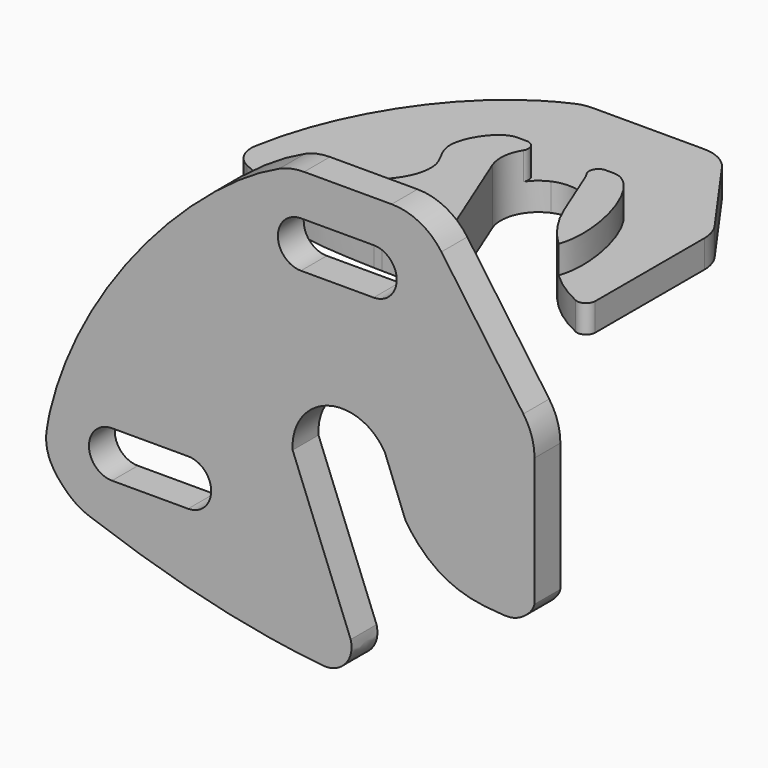
from build123d import *

# Parameters (mm, degrees)
F1_DEPTH    = 3
F2_DEPTH    = 6
F3_T1_DEPTH = 9.5721041615
F3_T3_DEPTH = 10.6008199663
F3_T5_DEPTH = 13.4715090396
F5_DEPTH    = 3.5
F6_R        = 6.6


# Not quite as in the source:
# - a fillet or chamfer that OpenCascade refuses, or shapes differently, is made with other operations: its cross-section is extruded or revolved along the edge and cut away or added


with BuildPart() as f1:
    # F0 (on Top) → F1 (new body)
    with BuildSketch(Plane.XY):
        with BuildLine():
            Line((10.45310308, 40.5577271794), (4.2537174463, 49.2922064861))
            ThreePointArc((4.2537174463, 49.2922064861), (2.8274809851, 50.5309572011), (0.9918162896, 50.9770389232))
            Line((0.9918162896, 50.9770389232), (-11.1394110977, 50.9770389232))
            ThreePointArc((-11.1394110977, 50.9770389232), (-11.971760899, 50.8894798248), (-12.7676708013, 50.6306358273))
            add(Edge.make_bspline(
                [(-29.0087616808, 27.7205901484), (-27.4187770892, 36.9581566811), (-21.4067194111, 46.7805628451), (-12.7676708013, 50.6306358273)],
                knots=[2.2635349129, 2.2635349129, 2.2635349129, 2.2635349129, 29.9811081227, 29.9811081227, 29.9811081227, 29.9811081227], degree=3))
            ThreePointArc((-29.0087616808, 27.7205901484), (-28.7134700585, 25.8268482821), (-27.3319649166, 24.4983532911))
            add(Edge.make_bspline(
                [(-27.3319649166, 24.4983532911), (-21.9405178356, 21.9555285826), (-18.2546260968, 21.2787347002), (-10.8634286016, 21.0598215648)],
                knots=[2.2151277371, 2.2151277371, 2.2151277371, 2.2151277371, 21.0948867648, 21.0948867648, 21.0948867648, 21.0948867648], degree=3))
            ThreePointArc((-10.8634286016, 21.0598215648), (-13.1384704579, 22.9593681642), (-12.6555627212, 25.8835591376))
            add(Edge.make_bspline(
                [(-8.9445100778, 38.260217756), (-10.7857445501, 38.3745139324), (-13.9860512104, 33.4519520511), (-10.6280428717, 30.4447296599), (-11.5734467469, 27.2133998528), (-12.6555627212, 25.8835591376)],
                knots=[0, 0, 0, 0, 0.371058298, 0.6724870623, 1, 1, 1, 1], degree=3))
            Line((-8.9445100778, 38.260217756), (-5.4481702034, 38.260217756))
            ThreePointArc((-5.4481702034, 38.260217756), (-3.7885215093, 38.6125725889), (-2.1288728152, 38.260217756))
            Line((-2.1288728152, 38.260217756), (1.3674670593, 38.260217756))
            add(Edge.make_bspline(
                [(5.8108489029, 25.2381619066), (7.2972377823, 29.2682433996), (4.5647696354, 38.260217756), (1.3674670593, 38.260217756)],
                knots=[0, 0, 0, 0, 13.7592725372, 13.7592725372, 13.7592725372, 13.7592725372], degree=3))
            ThreePointArc((5.8108489029, 25.2381619066), (8.3264404263, 23.3377486264), (11.1912019233, 22.0213471249))
            Line((11.1912019233, 22.0213471249), (11.1912019233, 38.2425596166))
            ThreePointArc((11.1912019233, 38.2425596166), (11.0022125915, 39.4575483765), (10.45310308, 40.5577271794))
        make_face()
    extrude(amount=F1_DEPTH)

    # F0 (on Top) → F2 (join)
    with BuildSketch(Plane.XY):
        with BuildLine():
            ThreePointArc((-12.6555627212, 25.8835591376), (-13.1384704579, 22.9593681642), (-10.8634286016, 21.0598215648))
            add(Edge.make_bspline(
                [(-10.8634286016, 21.0598215648), (-10.5727766997, 21.0512130112), (-10.2763949805, 21.0433125162), (-9.9739544094, 21.0360344499)],
                knots=[21.0948867648, 21.0948867648, 21.0948867648, 21.0948867648, 21.8373155625, 21.8373155625, 21.8373155625, 21.8373155625], degree=3))
            add(Edge.make_bspline(
                [(-9.9739544094, 21.0360344499), (-7.8814737991, 20.9856800532), (-5.4989697359, 20.9651199081), (-2.7174725462, 20.9459951911)],
                knots=[21.8373155625, 21.8373155625, 21.8373155625, 21.8373155625, 26.9739209391, 26.9739209391, 26.9739209391, 26.9739209391], degree=3))
            Line((-2.7174725462, 20.9459951911), (-7.5770430185, 33.0005098931))
            ThreePointArc((-7.5770430185, 33.0005098931), (-7.5749144289, 36.0603341373), (-5.4481702034, 38.260217756))
            Line((-5.4481702034, 38.260217756), (-8.9445100778, 38.260217756))
            add(Edge.make_bspline(
                [(-8.9445100778, 38.260217756), (-10.7857445501, 38.3745139324), (-13.9860512104, 33.4519520511), (-10.6280428717, 30.4447296599), (-11.5734467469, 27.2133998528), (-12.6555627212, 25.8835591376)],
                knots=[0, 0, 0, 0, 0.371058298, 0.6724870623, 1, 1, 1, 1], degree=3))
        make_face()
        with BuildLine():
            ThreePointArc((2.274153499, 30.4138629783), (3.7616023103, 27.6340666941), (5.8108489029, 25.2381619066))
            add(Edge.make_bspline(
                [(5.8108489029, 25.2381619066), (7.2972377823, 29.2682433996), (4.5647696354, 38.260217756), (1.3674670593, 38.260217756)],
                knots=[0, 0, 0, 0, 13.7592725372, 13.7592725372, 13.7592725372, 13.7592725372], degree=3))
            Line((1.3674670593, 38.260217756), (-2.1288728152, 38.260217756))
            ThreePointArc((-2.1288728152, 38.260217756), (-0.8497607567, 37.3648907946), (0, 36.0550645915))
            Line((0, 36.0550645915), (2.274153499, 30.4138629783))
        make_face()
    extrude(amount=F2_DEPTH)

    # F3: fillet of radius 1 on 4 edges, made by hand

    # F3_s2 → F3_t1 (cut)
    with BuildSketch(Plane.XY.offset(3)):
        with BuildLine():
            ThreePointArc((0.499968819, 38.260617756), (-0.3772452667, 37.7413074811), (-0.3438640289, 36.7224486062))
            Line((-0.3438640289, 36.7224486062), (-0.4282473137, 36.6686862987))
            ThreePointArc((-0.4282473137, 36.6686862987), (-1.1882692191, 37.5471857074), (-2.1695250121, 38.1687938896))
            Line((-2.1695250121, 38.1687938896), (-2.1288728152, 38.3602723635))
            ThreePointArc((-2.1288728152, 38.3602723635), (-0.8144519981, 38.3602723635), (0.499968819, 38.3606723635))
            Line((0.499968819, 38.3606723635), (0.499968819, 38.260617756))
        make_face()
        with BuildLine():
            ThreePointArc((-7.2331789896, 36.7224486062), (-7.1997977518, 37.7413074811), (-8.0770118375, 38.260617756))
            Line((-8.0770118375, 38.260617756), (-8.0770118375, 38.3606723635))
            ThreePointArc((-8.0770118375, 38.3606723635), (-6.7625910205, 38.3602723635), (-5.4481702034, 38.3602723635))
            Line((-5.4481702034, 38.3602723635), (-5.4075180064, 38.1687938896))
            ThreePointArc((-5.4075180064, 38.1687938896), (-6.3887737994, 37.5471857074), (-7.1487957048, 36.6686862987))
            Line((-7.1487957048, 36.6686862987), (-7.2331789896, 36.7224486062))
        make_face()
    extrude(amount=F3_T1_DEPTH, mode=Mode.SUBTRACT)

    # F3_s4 → F3_t3 (cut)
    with BuildSketch(Plane.XY.offset(-3.8004099831)):
        with BuildLine():
            ThreePointArc((11.1916019233, 23.4885064568), (10.7325048788, 22.646896313), (9.7763486506, 22.577304662))
            Line((9.7763486506, 22.577304662), (9.7349195602, 22.4861844826))
            ThreePointArc((9.7349195602, 22.4861844826), (10.4399749968, 22.187945003), (11.1594664861, 21.9264149456))
            Line((11.1594664861, 21.9264149456), (11.2912981602, 22.0213471249))
            ThreePointArc((11.2912981602, 22.0213471249), (11.2912981602, 22.7549267908), (11.2916981602, 23.4885064568))
            Line((11.2916981602, 23.4885064568), (11.1916019233, 23.4885064568))
        make_face()
    extrude(amount=F3_T3_DEPTH, mode=Mode.SUBTRACT)

    # F3_s6 → F3_t5 (cut)
    with BuildSketch(Plane.XY.offset(-3.7357545198)):
        with BuildLine():
            ThreePointArc((-4.2117376788, 20.9564645154), (-3.3765423085, 21.3940842593), (-3.2756110194, 22.3315677107))
            Line((-3.2756110194, 22.3315677107), (-3.1827802011, 22.36899086))
            ThreePointArc((-3.1827802011, 22.36899086), (-2.9038964588, 21.6761298214), (-2.6246417279, 20.9834183404))
            Line((-2.6246417279, 20.9834183404), (-2.7181607194, 20.845907333))
            ThreePointArc((-2.7181607194, 20.845907333), (-3.4653294824, 20.8511683916), (-4.2125195264, 20.8563773452))
            Line((-4.2125195264, 20.8563773452), (-4.2117376788, 20.9564645154))
        make_face()
    extrude(amount=F3_T5_DEPTH, mode=Mode.SUBTRACT)


with BuildPart() as f5:
    # F4 (on Front) → F5 (new body)
    with BuildSketch(Plane.XZ):
        with BuildLine():
            Line((14.1390746722, 23.0584476056), (0, 23.0584476056))
            add(Edge.make_bspline(
                [(0, 23.0584476056), (-8.4535141542, 20.1880769287), (-22.7127716179, 6.3917831067), (-26.3238836487, -8.8859928317)],
                knots=[0, 0, 0, 0, 41.3931651992, 41.3931651992, 41.3931651992, 41.3931651992], degree=3))
            add(Edge.make_bspline(
                [(-26.3238836487, -8.8859928317), (-26.509068396, -10.5526585131), (-28.0831411124, -13.2378456251), (-23.0831411124, -16.9415476647)],
                knots=[0, 0, 0, 0, 8.6829934846, 8.6829934846, 8.6829934846, 8.6829934846], degree=3))
            add(Edge.make_bspline(
                [(-23.0831411124, -16.9415476647), (-14.6371967644, -20.0166199929), (-6.0209512889, -22.4115496181), (3.1183243935, -23.3199736464)],
                knots=[0, 0, 0, 0, 26.9666666954, 26.9666666954, 26.9666666954, 26.9666666954], degree=3))
            add(Edge.make_bspline(
                [(3.1183243935, -23.3199736464), (4.9657123966, -23.6327832907), (6.820880084, -21.9836037196), (6.285587075, -19.8813614394)],
                knots=[0, 0, 0, 0, 4.6749980538, 4.6749980538, 4.6749980538, 4.6749980538], degree=3))
            Line((6.285587075, -19.8813614394), (0, -3.8729886569))
            ThreePointArc((0, -3.8729886569), (3.8002485038, 1.6052218538), (9.9970226848, -0.8549953803))
            Line((9.9970226848, -0.8549953803), (12.2130213435, -6.5945704318))
            add(Edge.make_bspline(
                [(26.1941587867, -10.0408689125), (25.9735344786, -10.923362591), (24.2632095256, -12.299581949), (21.6631683272, -12.0788543535), (15.4348382149, -11.5686364052), (12.2130213435, -6.5945704318)],
                knots=[0, 0, 0, 0, 0.2502484637, 0.4869890089, 1, 1, 1, 1], degree=3))
            Line((26.1941587867, -10.0408689125), (26.1941587867, 5.9918376473))
            Line((26.1941587867, 5.9918376473), (14.1390746722, 23.0584476056))
        make_face()
        with BuildLine():
            ThreePointArc((-19.5646238201, -13.1452520691), (-22.0646238201, -10.6452520691), (-19.5646238201, -8.1452520691))
            Line((-19.5646238201, -8.1452520691), (-11.3238848311, -8.1452520691))
            ThreePointArc((-11.3238848311, -8.1452520691), (-8.8238848311, -10.6452520691), (-11.3238848311, -13.1452520691))
            Line((-11.3238848311, -13.1452520691), (-19.5646238201, -13.1452520691))
        make_face(mode=Mode.SUBTRACT)
        with BuildLine():
            ThreePointArc((0.8983360527, 13.5214118386), (-1.6016639473, 16.0214118386), (0.8983360527, 18.5214118386))
            Line((0.8983360527, 18.5214118386), (8.7687045865, 18.5214118386))
            ThreePointArc((8.7687045865, 18.5214118386), (11.2687045865, 16.0214118386), (8.7687045865, 13.5214118386))
            Line((8.7687045865, 13.5214118386), (0.8983360527, 13.5214118386))
        make_face(mode=Mode.SUBTRACT)
    extrude(amount=F5_DEPTH)

    # F6
    f6_edges = [f5.edges().sort_by_distance(p)[0] for p in [
        (0, -1.75, 23.058448),
        (14.139075, -1.75, 23.058448),
        (26.194159, -1.75, 5.991838),
        (-23.083141, -1.75, -16.941548),
    ]]
    fillet(f6_edges, radius=F6_R)


solid = Compound([f1.part, f5.part])
